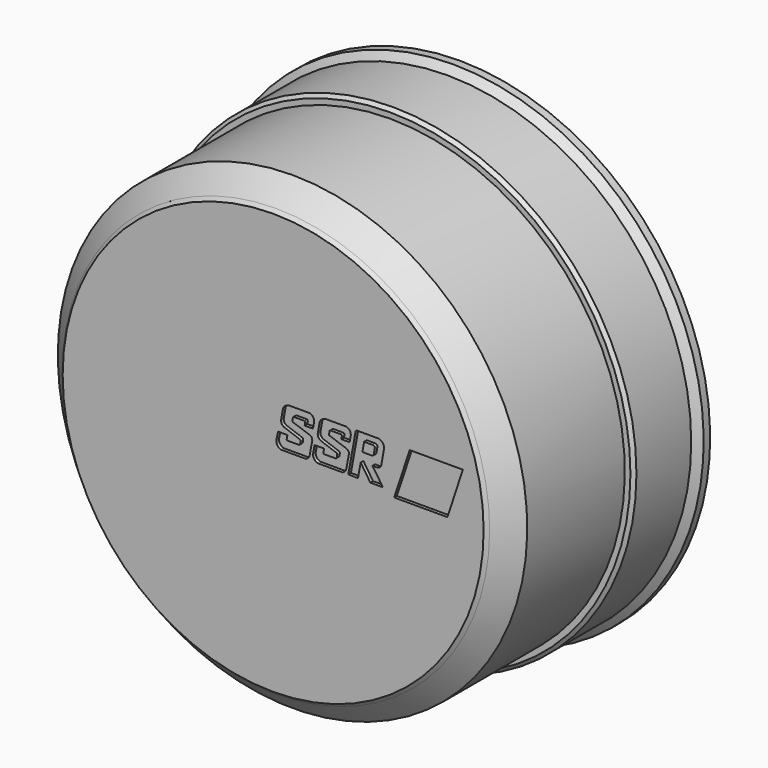
from build123d import *

# Parameters (mm, degrees)
F2_SIZE  = 0.508
F3_SIZE  = 3.175
F4_R     = 32.512
F5_DEPTH = 0.508
F6_SIZE  = 0.50799
F7_SIZE  = 1


# Not quite as in the source:
# - a fillet or chamfer is up to 0.001 mm smaller than in the source, because OpenCascade refuses the exact size


with BuildPart() as f1:
    # F0 (on Right) → F1 (revolve)
    with BuildSketch(Plane.YZ):
        Polygon((0, 35.687), (0, 0), (3.175, 0), (3.175, 31.75), (22.987, 31.75), (22.987, 35.04946), (34.925, 35.04946), (34.925, 38.1), (33.69056, 38.1), (32.639, 37.04844), (21.717, 37.04844), (21.717, 35.687), align=None)
    revolve(axis=Axis((0, 1.5875, 0), (0, -1, 0)))

    # F2
    f2_edges = [f1.edges().sort_by_distance(p)[0] for p in [
        (0, 21.717, -37.04844),
        (0, 22.987, -31.75),
    ]]
    chamfer(f2_edges, length=F2_SIZE)

    # F3
    f3_edges = [f1.edges().sort_by_distance(p)[0] for p in [
        (0, 0, -35.687),
    ]]
    chamfer(f3_edges, length=F3_SIZE)

    # F4 (on face) → F5 (join)
    with BuildSketch(Plane.XZ):
        Circle(F4_R)
        with BuildLine():
            ThreePointArc((1.509855967, 6.4400210977), (1.8937491355, 6.9297046378), (2.4878198747, 7.1147556882))
            Line((2.4878198747, 7.1147556882), (5.5111409165, 7.1147556882))
            ThreePointArc((5.5111409165, 7.1147556882), (6.0757301057, 6.7551068727), (6.2165134586, 6.1006695032))
            Line((6.2165134586, 6.1006695032), (6.0470685713, 5.1900157705))
            Line((6.0470685713, 5.1900157705), (4.7878890863, 5.1900157705))
            Line((4.7878890863, 5.1900157705), (4.8664845526, 5.5916425772))
            ThreePointArc((4.8664845526, 5.5916425772), (4.836723562, 5.7383814637), (4.7118113372, 5.8209341951))
            Line((4.7118113372, 5.8209341951), (3.1333588995, 5.8209341951))
            ThreePointArc((3.1333588995, 5.8209341951), (3.0458218752, 5.7703284959), (3.0000514816, 5.6801689789))
            Line((3.0000514816, 5.6801689789), (2.9189020861, 5.2375365049))
            ThreePointArc((2.9189020861, 5.2375365049), (2.9425937197, 5.1281238685), (3.0369379092, 5.0678611733))
            Line((3.0369379092, 5.0678611733), (5.5451882072, 4.1973507032))
            ThreePointArc((5.5451882072, 4.1973507032), (5.8744055755, 3.9176753087), (5.9288027696, 3.4891390242))
            Line((5.9288027696, 3.4891390242), (5.5599426851, 1.5120476019))
            ThreePointArc((5.5599426851, 1.5120476019), (5.3557662432, 1.0797199091), (4.9655372277, 0.8034653729))
            Line((4.9655372277, 0.8034653729), (1.2082514586, 0.8034653729))
            ThreePointArc((1.2082514586, 0.8034653729), (0.6584047868, 1.1902455436), (0.4886787001, 1.8407248426))
            Line((0.4886787001, 1.8407248426), (0.7345082122, 3.0832483899))
            Line((0.7345082122, 3.0832483899), (2.1749762818, 3.0832483899))
            Line((2.1749762818, 3.0832483899), (2.0602140576, 2.5084333029))
            ThreePointArc((2.0602140576, 2.5084333029), (2.0616584556, 2.3899178369), (2.1645433735, 2.3310731631))
            Line((2.1645433735, 2.3310731631), (3.9138016291, 2.3310731631))
            ThreePointArc((3.9138016291, 2.3310731631), (4.0417506777, 2.3951715526), (4.1066328995, 2.5227249134))
            Line((4.1066328995, 2.5227249134), (4.1656503454, 2.9063397087))
            ThreePointArc((4.1656503454, 2.9063397087), (4.1228902349, 3.0507674018), (4.0033520199, 3.1424101908))
            Line((4.0033520199, 3.1424101908), (1.6647774028, 3.9686574601))
            ThreePointArc((1.6647774028, 3.9686574601), (1.2895839844, 4.3349438035), (1.2147676898, 4.8539219424))
            Line((1.2147676898, 4.8539219424), (1.509855967, 6.4400210977))
        make_face(mode=Mode.SUBTRACT)
        with BuildLine():
            Line((6.0626888962, 1.8407248426), (6.3085184083, 3.0832483899))
            Line((6.3085184083, 3.0832483899), (7.748986478, 3.0832483899))
            Line((7.748986478, 3.0832483899), (7.6342242537, 2.5084333029))
            ThreePointArc((7.6342242537, 2.5084333029), (7.6356686517, 2.3899178369), (7.7385535697, 2.3310731631))
            Line((7.7385535697, 2.3310731631), (9.4878118252, 2.3310731631))
            ThreePointArc((9.4878118252, 2.3310731631), (9.6157608738, 2.3951715526), (9.6806430956, 2.5227249134))
            Line((9.6806430956, 2.5227249134), (9.7396605415, 2.9063397087))
            ThreePointArc((9.7396605415, 2.9063397087), (9.696900431, 3.0507674018), (9.5773622161, 3.1424101908))
            Line((9.5773622161, 3.1424101908), (7.2387875989, 3.9686574601))
            ThreePointArc((7.2387875989, 3.9686574601), (6.8635941806, 4.3349438035), (6.788777886, 4.8539219424))
            Line((6.788777886, 4.8539219424), (7.0838661632, 6.4400210977))
            ThreePointArc((7.0838661632, 6.4400210977), (7.4677593317, 6.9297046378), (8.0618300708, 7.1147556882))
            Line((8.0618300708, 7.1147556882), (11.0851511126, 7.1147556882))
            ThreePointArc((11.0851511126, 7.1147556882), (11.6497403019, 6.7551068727), (11.7905236548, 6.1006695032))
            Line((11.7905236548, 6.1006695032), (11.6210787675, 5.1900157705))
            Line((11.6210787675, 5.1900157705), (10.3618992824, 5.1900157705))
            Line((10.3618992824, 5.1900157705), (10.4404947488, 5.5916425772))
            ThreePointArc((10.4404947488, 5.5916425772), (10.4107337581, 5.7383814637), (10.2858215333, 5.8209341951))
            Line((10.2858215333, 5.8209341951), (8.7073690956, 5.8209341951))
            ThreePointArc((8.7073690956, 5.8209341951), (8.6198320713, 5.7703284959), (8.5740616778, 5.6801689789))
            Line((8.5740616778, 5.6801689789), (8.4929122822, 5.2375365049))
            ThreePointArc((8.4929122822, 5.2375365049), (8.5166039159, 5.1281238685), (8.6109481053, 5.0678611733))
            Line((8.6109481053, 5.0678611733), (11.1191984033, 4.1973507032))
            ThreePointArc((11.1191984033, 4.1973507032), (11.4484157717, 3.9176753087), (11.5028129658, 3.4891390242))
            Line((11.5028129658, 3.4891390242), (11.1339528812, 1.5120476019))
            ThreePointArc((11.1339528812, 1.5120476019), (10.9297764394, 1.0797199091), (10.5395474238, 0.8034653729))
            Line((10.5395474238, 0.8034653729), (6.7822616547, 0.8034653729))
            ThreePointArc((6.7822616547, 0.8034653729), (6.232414983, 1.1902455436), (6.0626888962, 1.8407248426))
        make_face(mode=Mode.SUBTRACT)
        with BuildLine():
            Line((15.0836538523, 3.1598797068), (16.7005891971, 0.8034653729))
            Line((16.7005891971, 0.8034653729), (14.781959715, 0.8034653729))
            Line((14.781959715, 0.8034653729), (13.311708346, 3.0348771252))
            Line((13.311708346, 3.0348771252), (12.8936721012, 0.8034653729))
            Line((12.8936721012, 0.8034653729), (11.4200627431, 0.8034653729))
            Line((11.4200627431, 0.8034653729), (12.5739071518, 7.1147556882))
            Line((12.5739071518, 7.1147556882), (15.9580335021, 7.1147556882))
            ThreePointArc((15.9580335021, 7.1147556882), (16.6617692136, 6.7173463158), (16.8489553034, 5.9311278164))
            Line((16.8489553034, 5.9311278164), (16.4579637349, 3.7548521068))
            ThreePointArc((16.4579637349, 3.7548521068), (16.2392824666, 3.3522910872), (15.8235244453, 3.1598797068))
            Line((15.8235244453, 3.1598797068), (15.0836538523, 3.1598797068))
        make_face(mode=Mode.SUBTRACT)
        Polygon((26.1573679745, 7.1147556882), (28.8369659559, 7.1147556882), (26.4996811748, 0), (23.7947255373, 0), (21.1136136204, 0), (18.4020102024, 0), (20.7625944167, 7.1147556882), (23.4577525407, 7.1147556882), align=None, mode=Mode.SUBTRACT)
        with BuildLine():
            Line((15.154549852, 5.9737088159), (13.8270081952, 5.9737088159))
            Line((13.8270081952, 5.9737088159), (13.5664623231, 4.509691149))
            Line((13.5664623231, 4.509691149), (14.9684455246, 4.509691149))
            ThreePointArc((14.9684455246, 4.509691149), (15.1889852841, 4.5698286448), (15.3071191162, 4.7655291855))
            Line((15.3071191162, 4.7655291855), (15.4472859576, 5.6212851778))
            ThreePointArc((15.4472859576, 5.6212851778), (15.3812525761, 5.8642259453), (15.154549852, 5.9737088159))
        make_face()
    extrude(amount=F5_DEPTH)

    # F6 (size 0.508 in the source; OpenCascade refuses exactly that, so slightly less here)
    f6_edges = [f1.edges().sort_by_distance(p)[0] for p in [
        (0, 12.446, 35.687),
        (-32.512, -0.508, 0),
    ]]
    chamfer(f6_edges, length=F6_SIZE)

    # F7
    f7_edges = [f1.edges().sort_by_distance(p)[0] for p in [
        (0, 34.925, -35.04946),
    ]]
    chamfer(f7_edges, length=F7_SIZE)


solid = f1.part
